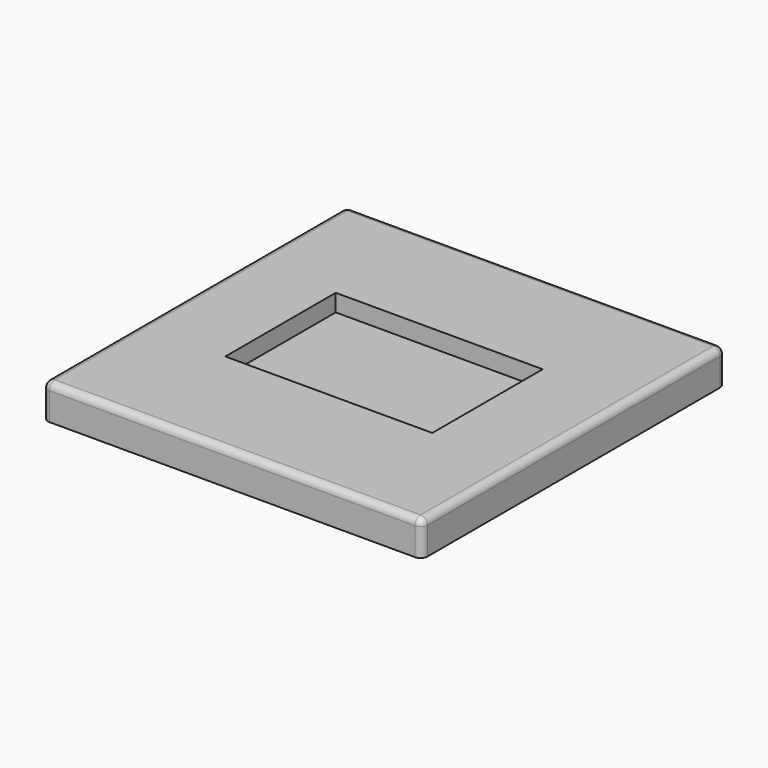
from build123d import *

# Parameters (mm, degrees)
F0_W         = 550
F0_H         = 550
F1_DEPTH     = 50
F2_R         = 10
F3_T1_DEPTH  = 65
F3_S5_W      = 10
F3_S5_H      = 10
F3_T6_DEPTH  = 10
F3_S11_W     = 10
F3_S11_H     = 10
F3_T12_DEPTH = 10
F3_S17_W     = 10
F3_S17_H     = 10
F3_T18_DEPTH = 10
F3_S23_W     = 10
F3_S23_H     = 10
F3_T24_DEPTH = 10
F4_W         = 300
F4_H         = 200
F5_DEPTH     = 25


# Not quite as in the source:
# - a fillet or chamfer that OpenCascade refuses, or shapes differently, is made with other operations: its cross-section is extruded or revolved along the edge and cut away or added


with BuildPart() as f1:
    # F0 (on Top) → F1 (new body)
    with BuildSketch(Plane.XY):
        Rectangle(F0_W, F0_H)
    extrude(amount=F1_DEPTH)

    # F2
    f2_edges = [f1.edges().sort_by_distance(p)[0] for p in [
        (0, -275, 50),
        (275, 0, 50),
        (0, 275, 50),
        (-275, 0, 50),
    ]]
    fillet(f2_edges, radius=F2_R)

    # F3: fillet of radius 10 on 4 edges, made by hand

    # F3_s2 → F3_t1 (cut)
    with BuildSketch(Plane.XY.offset(-25)):
        with BuildLine():
            ThreePointArc((275, -265), (272.0710678119, -272.0710678119), (265, -275))
            Line((265, -275), (275, -275))
            Line((275, -275), (275, -265))
        make_face()
        with BuildLine():
            ThreePointArc((-265, -275), (-272.0710678119, -272.0710678119), (-275, -265))
            Line((-275, -265), (-275, -275))
            Line((-275, -275), (-265, -275))
        make_face()
        with BuildLine():
            ThreePointArc((275, 265), (272.0710678119, 272.0710678119), (265, 275))
            Line((265, 275), (275, 275))
            Line((275, 275), (275, 265))
        make_face()
        with BuildLine():
            ThreePointArc((-265, 275), (-272.0710678119, 272.0710678119), (-275, 265))
            Line((-275, 265), (-275, 275))
            Line((-275, 275), (-265, 275))
        make_face()
    extrude(amount=F3_T1_DEPTH, mode=Mode.SUBTRACT)


with BuildPart() as f3_tool4:
    # F3_s5 → F3_t6 (new body)
    with BuildSketch(Plane.XZ.offset(-265)):
        with Locations((-270, 45)):
            Rectangle(F3_S5_W, F3_S5_H)
    extrude(amount=-F3_T6_DEPTH)

    # F3_s7 → F3_t8 (revolve, cut)
    with BuildSketch(Plane(origin=(-265, 265, 40), x_dir=(0.7071067812, 0, -0.7071067812), z_dir=(0.7071067812, 0, 0.7071067812))):
        with BuildLine():
            ThreePointArc((0, -10), (10, 0), (0, 10))
            Line((0, 10), (0, -10))
        make_face()
    revolve(axis=Axis((-265, 265, 40), (0, 1, 0)), mode=Mode.SUBTRACT)


with BuildPart() as f1_1:
    add(f1.part)

    # F3_t3: cut F3_tool4
    add(f3_tool4.part, mode=Mode.SUBTRACT)


with BuildPart() as f3_tool10:
    # F3_s11 → F3_t12 (new body)
    with BuildSketch(Plane.YZ.offset(265)):
        with Locations((270, 45)):
            Rectangle(F3_S11_W, F3_S11_H)
    extrude(amount=F3_T12_DEPTH)

    # F3_s13 → F3_t14 (revolve, cut)
    with BuildSketch(Plane(origin=(265, 265, 40), x_dir=(0, -0.7071067812, -0.7071067812), z_dir=(0, -0.7071067812, 0.7071067812))):
        with BuildLine():
            ThreePointArc((0, -10), (10, 0), (0, 10))
            Line((0, 10), (0, -10))
        make_face()
    revolve(axis=Axis((265, 265, 40), (1, 0, 0)), mode=Mode.SUBTRACT)


with BuildPart() as f1_2:
    add(f1_1.part)

    # F3_t9: cut F3_tool10
    add(f3_tool10.part, mode=Mode.SUBTRACT)


with BuildPart() as f3_tool16:
    # F3_s17 → F3_t18 (new body)
    with BuildSketch(Plane.XZ.offset(265)):
        with Locations((-270, 45)):
            Rectangle(F3_S17_W, F3_S17_H)
    extrude(amount=F3_T18_DEPTH)

    # F3_s19 → F3_t20 (revolve, cut)
    with BuildSketch(Plane(origin=(-265, -265, 40), x_dir=(0.7071067812, 0, -0.7071067812), z_dir=(-0.7071067812, 0, -0.7071067812))):
        with BuildLine():
            ThreePointArc((0, -10), (10, 0), (0, 10))
            Line((0, 10), (0, -10))
        make_face()
    revolve(axis=Axis((-265, -265, 40), (0, -1, 0)), mode=Mode.SUBTRACT)


with BuildPart() as f1_3:
    add(f1_2.part)

    # F3_t15: cut F3_tool16
    add(f3_tool16.part, mode=Mode.SUBTRACT)


with BuildPart() as f3_tool22:
    # F3_s23 → F3_t24 (new body)
    with BuildSketch(Plane.YZ.offset(265)):
        with Locations((-270, 45)):
            Rectangle(F3_S23_W, F3_S23_H)
    extrude(amount=F3_T24_DEPTH)

    # F3_s25 → F3_t26 (revolve, cut)
    with BuildSketch(Plane(origin=(265, -265, 40), x_dir=(0, 0.7071067812, -0.7071067812), z_dir=(0, -0.7071067812, -0.7071067812))):
        with BuildLine():
            ThreePointArc((0, -10), (10, 0), (0, 10))
            Line((0, 10), (0, -10))
        make_face()
    revolve(axis=Axis((265, -265, 40), (1, 0, 0)), mode=Mode.SUBTRACT)


with BuildPart() as f1_4:
    add(f1_3.part)

    # F3_t21: cut F3_tool22
    add(f3_tool22.part, mode=Mode.SUBTRACT)

    # F4 (on face) → F5 (cut)
    with BuildSketch(Plane.XY.offset(50)):
        Rectangle(F4_W, F4_H)
    extrude(amount=-F5_DEPTH, mode=Mode.SUBTRACT)


solid = f1_4.part
